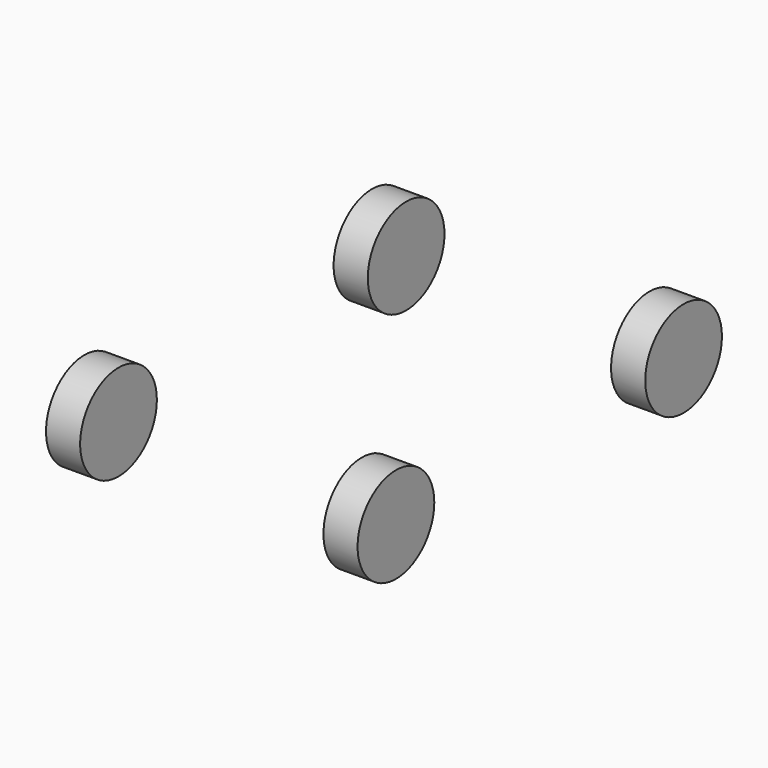
from build123d import *

# Parameters (mm, degrees)
F2_R     = 400
F3_DEPTH = 285


# Not quite as in the source:
# - a pattern or mirror of a feature is missing from the dataset's text; its kind, count and spacing are read off the source's solid


with BuildPart() as f3:
    # F2 (on offset) → F3 (new body)
    with BuildSketch(Plane.YZ.offset(1300)):
        with Locations((0, 400)):
            Circle(F2_R)
    extrude(amount=-F3_DEPTH)


with BuildPart() as f3b:
    # F2 (on offset) → F3, piece 2 (new body)
    with BuildSketch(Plane.YZ.offset(1300)):
        with Locations((3000, 400)):
            Circle(F2_R)
    extrude(amount=-F3_DEPTH)


with BuildPart() as f3_copies_1:
    # F3_copies: instance of F3
    add(f3.part.mirror(Plane(origin=(0, 0, 0), x_dir=(0, 0, -1), z_dir=(-1, 0, 0))))


with BuildPart() as f3_2_copies_1:
    # F3_2_copies: instance of F3b
    add(f3b.part.mirror(Plane(origin=(0, 0, 0), x_dir=(0, 0, -1), z_dir=(-1, 0, 0))))


solid = Compound([f3.part, f3b.part, f3_copies_1.part, f3_2_copies_1.part])
